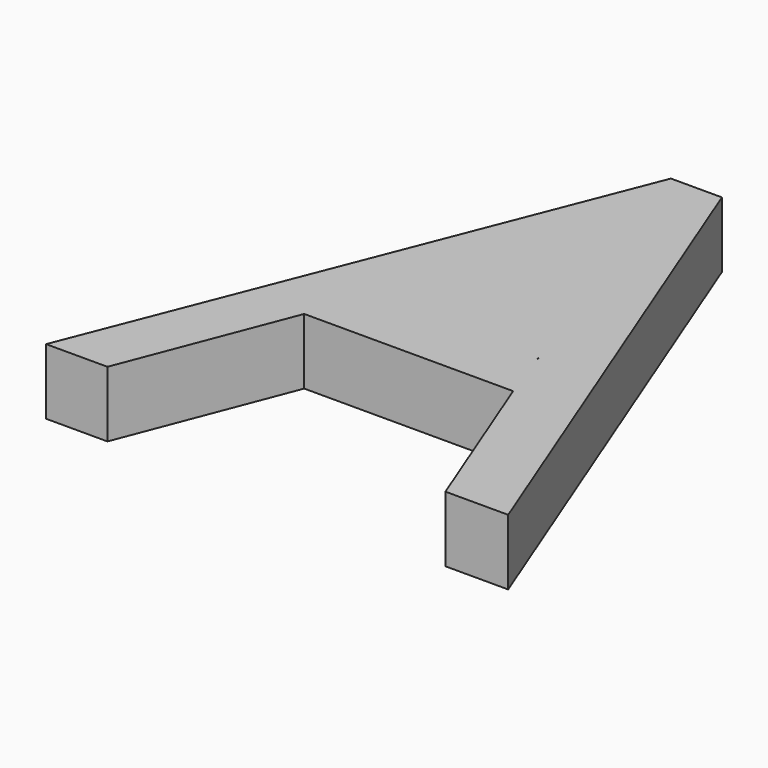
from build123d import *

# Parameters (mm, degrees)
F1_DEPTH = 25.4
F2_DEPTH = 25.4


with BuildPart() as f1:
    # F0 (on Top) → F1 (new body)
    with BuildSketch(Plane.XY):
        Polygon((-123.5604166667, 188.4609023112), (-203.2, -13.8571532443), (-179.4756944444, -13.8571532443), (-154.6930555556, 50.2161106446), (-73.9510416667, 50.2161106446), (-48.8597222222, -13.8571532443), (-24.60625, -13.8571532443), (-103.8489583333, 188.4609023112), align=None)
        Polygon((-81.5007686615, 67.9640099406), (-152.8517007828, 67.9640099406), (-152.8517007828, 106.1364486814), (-139.8437470198, 106.1364486814), (-139.8437470198, 137.258246541), (-127.1816492081, 137.258246541), (-127.1816492081, 169.5059537888), (-101.4676243067, 169.5059537888), (-101.4676243067, 137.258246541), (-90.7859355211, 137.258246541), (-90.7859355211, 106.1364486814), (-81.5007686615, 106.1364486814), (-81.5007686615, 72.0230385523), (-81.2270833333, 71.2945828668), (-81.5007686615, 71.2945828668), align=None, mode=Mode.SUBTRACT)
    extrude(amount=F1_DEPTH)

    # F0 (on Top) → F2 (join)
    with BuildSketch(Plane.XY):
        Polygon((-146.4027777778, 71.2945828668), (-81.5007686615, 71.2945828668), (-81.5007686615, 72.0230385523), (-94.3173888512, 106.1364486814), (-133.1894430727, 106.1364486814), align=None)
        with BuildLine():
            Line((-122.7225694444, 133.7362495335), (-133.1894430727, 106.1364486814))
            Line((-133.1894430727, 106.1364486814), (-94.3173888512, 106.1364486814))
            Line((-94.3173888512, 106.1364486814), (-104.6868055556, 133.7362495335))
            add(Edge.make_bspline(
                [(-104.6868055556, 133.7362495335), (-105.3399663206, 135.4420771625), (-105.9985985773, 137.258246541)],
                knots=[0, 0, 0, 0.1438042201, 0.1438042201, 0.1438042201], degree=2))
            Line((-105.9985985773, 137.258246541), (-121.4879183379, 137.258246541))
            add(Edge.make_bspline(
                [(-121.4879183379, 137.258246541), (-122.0888459048, 135.5136460237), (-122.7225694444, 133.7362495335)],
                knots=[0.8877261445, 0.8877261445, 0.8877261445, 1, 1, 1], degree=2))
        make_face()
        with BuildLine():
            Line((-127.1816492081, 169.5059537888), (-127.1816492081, 137.258246541))
            Line((-127.1816492081, 137.258246541), (-121.4879183379, 137.258246541))
            add(Edge.make_bspline(
                [(-114.0354166667, 162.7963189779), (-116.7365084044, 151.0524418574), (-121.4879183379, 137.258246541)],
                knots=[0, 0, 0, 0.8877261445, 0.8877261445, 0.8877261445], degree=2))
            add(Edge.make_bspline(
                [(-105.9985985773, 137.258246541), (-109.9200284094, 148.071535305), (-114.0354166667, 162.7963189779)],
                knots=[0.1438042201, 0.1438042201, 0.1438042201, 1, 1, 1], degree=2))
            Line((-105.9985985773, 137.258246541), (-101.4676243067, 137.258246541))
            Line((-101.4676243067, 137.258246541), (-101.4676243067, 169.5059537888))
            Line((-101.4676243067, 169.5059537888), (-127.1816492081, 169.5059537888))
        make_face()
        with BuildLine():
            Line((-139.8437470198, 137.258246541), (-139.8437470198, 106.1364486814))
            Line((-139.8437470198, 106.1364486814), (-133.1894430727, 106.1364486814))
            Line((-133.1894430727, 106.1364486814), (-122.7225694444, 133.7362495335))
            add(Edge.make_bspline(
                [(-121.4879183379, 137.258246541), (-122.0888459048, 135.5136460237), (-122.7225694444, 133.7362495335)],
                knots=[0.8877261445, 0.8877261445, 0.8877261445, 1, 1, 1], degree=2))
            Line((-121.4879183379, 137.258246541), (-127.1816492081, 137.258246541))
            Line((-127.1816492081, 137.258246541), (-139.8437470198, 137.258246541))
        make_face()
        Polygon((-152.8517007828, 106.1364486814), (-152.8517007828, 67.9640099406), (-81.5007686615, 67.9640099406), (-81.5007686615, 71.2945828668), (-146.4027777778, 71.2945828668), (-133.1894430727, 106.1364486814), (-139.8437470198, 106.1364486814), align=None)
        with BuildLine():
            Line((-104.6868055556, 133.7362495335), (-94.3173888512, 106.1364486814))
            Line((-94.3173888512, 106.1364486814), (-90.7859355211, 106.1364486814))
            Line((-90.7859355211, 106.1364486814), (-90.7859355211, 137.258246541))
            Line((-90.7859355211, 137.258246541), (-101.4676243067, 137.258246541))
            Line((-101.4676243067, 137.258246541), (-105.9985985773, 137.258246541))
            add(Edge.make_bspline(
                [(-104.6868055556, 133.7362495335), (-105.3399663206, 135.4420771625), (-105.9985985773, 137.258246541)],
                knots=[0, 0, 0, 0.1438042201, 0.1438042201, 0.1438042201], degree=2))
        make_face()
        Polygon((-94.3173888512, 106.1364486814), (-81.5007686615, 72.0230385523), (-81.5007686615, 106.1364486814), (-90.7859355211, 106.1364486814), align=None)
        with BuildLine():
            add(Edge.make_bspline(
                [(-114.0354166667, 162.7963189779), (-116.7365084044, 151.0524418574), (-121.4879183379, 137.258246541)],
                knots=[0, 0, 0, 0.8877261445, 0.8877261445, 0.8877261445], degree=2))
            Line((-121.4879183379, 137.258246541), (-105.9985985773, 137.258246541))
            add(Edge.make_bspline(
                [(-105.9985985773, 137.258246541), (-109.9200284094, 148.071535305), (-114.0354166667, 162.7963189779)],
                knots=[0.1438042201, 0.1438042201, 0.1438042201, 1, 1, 1], degree=2))
        make_face()
    extrude(amount=F2_DEPTH)


solid = f1.part
